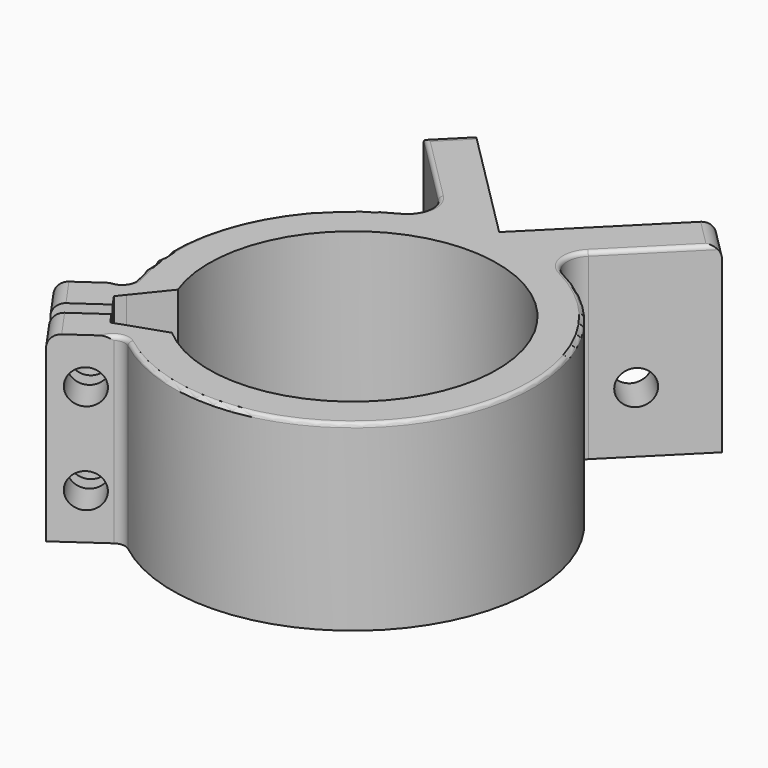
from build123d import *

# Parameters (mm, degrees)
F1_DEPTH      = 45
F2_R          = 4.25
F3_DEPTH      = 10
F4_R          = 4.25
F5_DEPTH      = 10
F6_R          = 4.25
F7_DEPTH      = 22
F9_DEPTH      = 3
F10_R         = 6
F11_T1_DEPTH  = 45
F11_T6_DEPTH  = 45
F11_T11_DEPTH = 50.6773888561
F11_T16_DEPTH = 56.3547777122
F11_T22_DEPTH = 50.6773888561
F11_T24_DEPTH = 24
F11_T26_DEPTH = 24
F11_T28_DEPTH = 25
F11_T30_DEPTH = 25
F12_T3_ANGLE  = 191.1142548037
F12_T6_ANGLE  = 120.6172934525
F12_T9_ANGLE  = 108.2560127517
F12_T12_DEPTH = 25.3616591831
F12_T15_DEPTH = 25.3616591831
F12_T18_ANGLE = 108.2560127517
F12_T21_ANGLE = 120.6172934336
F12_T24_ANGLE = 81.1142548036


# Not quite as in the source:
# - a fillet or chamfer that OpenCascade refuses, or shapes differently, is made with other operations: its cross-section is extruded or revolved along the edge and cut away or added


with BuildPart() as f1:
    # F0 (on Top) → F1 (new body)
    with BuildSketch(Plane.XY):
        with BuildLine():
            Line((29.6984848098, 29.6984848098), (0, 0))
            Line((0, 0), (-29.6984848098, 29.6984848098))
            Line((-29.6984848098, 29.6984848098), (-36.7695526217, 22.627416998))
            Line((-36.7695526217, 22.627416998), (-11.9950181388, -2.1471174849))
            ThreePointArc((-11.9950181388, -2.1471174849), (-39.7071381913, -24.9103714156), (-41.6303752657, -60.7213821032))
            ThreePointArc((-41.6303752657, -60.7213821032), (-40.7005404194, -62.9921096474), (-39.6469587391, -65.2081335788))
            Line((-39.6469587391, -65.2081335788), (-33.2920408775, -57.324366686))
            ThreePointArc((-33.2920408775, -57.324366686), (29.0798975723, -24.6380365095), (-22.9676650232, -72.0691034832))
            Line((-22.9676650232, -72.0691034832), (-32.5494925143, -75.3443658208))
            ThreePointArc((-32.5494925143, -75.3443658208), (-30.8274573358, -77.0923335738), (-29.011693666, -78.7427270775))
            ThreePointArc((-29.011693666, -78.7427270775), (39.2315391454, -66.0032458512), (11.9950181388, -2.1471174849))
            Line((11.9950181388, -2.1471174849), (36.7695526217, 22.627416998))
            Line((36.7695526217, 22.627416998), (29.6984848098, 29.6984848098))
        make_face()
        with BuildLine():
            ThreePointArc((-39.6469587391, -65.2081335788), (-40.7005404194, -62.9921096474), (-41.6303752657, -60.7213821032))
            Line((-41.6303752657, -60.7213821032), (-54.1929009582, -69.517757292))
            Line((-54.1929009582, -69.517757292), (-49.0307130311, -76.8901256906))
            Line((-49.0307130311, -76.8901256906), (-39.1915368437, -70.0006603545))
            Line((-39.1915368437, -70.0006603545), (-41.1990543709, -67.1336281995))
            Line((-41.1990543709, -67.1336281995), (-39.6469587391, -65.2081335788))
        make_face()
        with BuildLine():
            Line((-41.5742193585, -87.5391022664), (-29.011693666, -78.7427270775))
            ThreePointArc((-29.011693666, -78.7427270775), (-30.8274573358, -77.0923335738), (-32.5494925143, -75.3443658208))
            Line((-32.5494925143, -75.3443658208), (-34.8897135711, -76.1443006866))
            Line((-34.8897135711, -76.1443006866), (-36.8972310983, -73.2772685316))
            Line((-36.8972310983, -73.2772685316), (-46.7364072857, -80.1667338678))
            Line((-46.7364072857, -80.1667338678), (-41.5742193585, -87.5391022664))
        make_face()
    extrude(amount=F1_DEPTH)

    # F2 (on face) → F3 (cut, through all)
    with BuildSketch(Plane(origin=(0, 0, 0), x_dir=(-0.7071067812, -0.7071067812, 0), z_dir=(-0.7071067812, 0.7071067812, 0))):
        with Locations((-25.4, 15)):
            Circle(F2_R)
    extrude(amount=-F3_DEPTH, mode=Mode.SUBTRACT)

    # F4 (on face) → F5 (cut, through all)
    with BuildSketch(Plane(origin=(0, 0, 0), x_dir=(-0.7071067812, 0.7071067812, 0), z_dir=(0.7071067812, 0.7071067812, 0))):
        with Locations((25.4, 15)):
            Circle(F4_R)
    extrude(amount=-F5_DEPTH, mode=Mode.SUBTRACT)

    # F6 (on face) → F7 (cut, through all)
    with BuildSketch(Plane(origin=(27.4524247675, -39.206125712, 0), x_dir=(0.8191520443, 0.5735764364, 0), z_dir=(0.5735764364, -0.8191520443, 0))):
        with Locations((-76.5979670285, 33.75)):
            Circle(F6_R)
        with Locations((-76.5979670285, 11.25)):
            Circle(F6_R)
    extrude(amount=-F7_DEPTH, mode=Mode.SUBTRACT)

    # F8 (on face) → F9 (cut)
    with BuildSketch(Plane(origin=(14.8337431678, -21.1847807376, 0), x_dir=(-0.8191520443, -0.5735764364, 0), z_dir=(-0.5735764364, 0.8191520443, 0))):
        Polygon((83.5229670285, 37.7481506141), (76.5979670285, 41.7463012283), (69.6729670285, 37.7481506141), (69.6729670285, 29.7518493859), (76.5979670285, 25.7536987717), (83.5229670285, 29.7518493859), align=None)
        Polygon((76.5979670285, 19.2463012283), (69.6729670285, 15.2481506141), (69.6729670285, 7.2518493859), (76.5979670285, 3.2536987717), (83.5229670285, 7.2518493859), (83.5229670285, 15.2481506141), align=None)
    extrude(amount=-F9_DEPTH, mode=Mode.SUBTRACT)

    # F10
    f10_edges = [f1.edges().sort_by_distance(p)[0] for p in [
        (-11.995018, -2.147117, 22.5),
        (11.995018, -2.147117, 22.5),
    ]]
    fillet(f10_edges, radius=F10_R)

    # F11: fillet of radius 3 on 6 edges, made by hand

    # F11_s2 → F11_t1 (join)
    with BuildSketch(Plane.XY):
        with BuildLine():
            ThreePointArc((-27.3100924069, -80.1341550735), (-29.0764013889, -79.5036829691), (-30.8719515411, -80.0452936647))
            Line((-30.8719515411, -80.0452936647), (-29.011693666, -78.7427270775))
            ThreePointArc((-29.011693666, -78.7427270775), (-28.169485522, -79.4489489742), (-27.3100924069, -80.1341550735))
        make_face()
    extrude(amount=F11_T1_DEPTH)


with BuildPart() as f11_tool4:
    # F11_s5 → F11_t6 (new body)
    with BuildSketch(Plane.XY):
        with BuildLine():
            ThreePointArc((-42.3559079793, -58.6465035538), (-42.3675712465, -60.5219252298), (-43.4906331408, -62.0239486903))
            Line((-43.4906331408, -62.0239486903), (-41.6303752657, -60.7213821032))
            ThreePointArc((-41.6303752657, -60.7213821032), (-42.0059546205, -59.6884232108), (-42.3559079793, -58.6465035538))
        make_face()
    extrude(amount=F11_T6_DEPTH)

    split(bisect_by=Plane(origin=(-57.0727533731, -39.9627721382, 0), x_dir=(0, 0, 1), z_dir=(0.8191520443, 0.5735764364, 0)), keep=Keep.TOP)


with BuildPart() as f1_1:
    add(f1.part)

    # F11_t3: union F11_tool4
    add(f11_tool4.part)


with BuildPart() as f11_tool9:
    # F11_s10 → F11_t11 (new body)
    with BuildSketch(Plane.XY):
        with BuildLine():
            ThreePointArc((-42.3559079793, -58.6465035538), (-42.3675712465, -60.5219252298), (-43.4906331408, -62.0239486903))
            Line((-43.4906331408, -62.0239486903), (-41.6303752657, -60.7213821032))
            ThreePointArc((-41.6303752657, -60.7213821032), (-42.0059546205, -59.6884232108), (-42.3559079793, -58.6465035538))
        make_face()
    extrude(amount=F11_T11_DEPTH)

    split(bisect_by=Plane(origin=(-16.8404428161, -11.7918050066, 35.6081667412), x_dir=(-0.5735764364, 0.8191520443, 0), z_dir=(0.4095760221, 0.2867882182, -0.8660254038)), keep=Keep.TOP)


with BuildPart() as f1_2:
    add(f1_1.part)

    # F11_t8: union F11_tool9
    add(f11_tool9.part)


with BuildPart() as f11_tool14:
    # F11_s15 → F11_t16 (new body)
    with BuildSketch(Plane.XY.offset(-5.6773888561)):
        with BuildLine():
            ThreePointArc((-42.3559079793, -58.6465035538), (-42.3675712465, -60.5219252298), (-43.4906331408, -62.0239486903))
            Line((-43.4906331408, -62.0239486903), (-41.6303752657, -60.7213821032))
            ThreePointArc((-41.6303752657, -60.7213821032), (-42.0059546205, -59.6884232108), (-42.3559079793, -58.6465035538))
        make_face()
    extrude(amount=F11_T16_DEPTH)

    split(bisect_by=Plane(origin=(-24.8212657152, -17.3800373617, 52.4831667412), x_dir=(-0.5735764364, 0.8191520443, 0), z_dir=(0.4095760221, 0.2867882182, -0.8660254038)), keep=Keep.TOP)

    split(bisect_by=Plane(origin=(-8.8596199171, -6.2035726516, -18.7331667412), x_dir=(-0.5735764364, 0.8191520443, 0), z_dir=(0.4095760221, 0.2867882182, 0.8660254038)), keep=Keep.TOP)


with BuildPart() as f1_3:
    add(f1_2.part)

    # F11_t13: union F11_tool14
    add(f11_tool14.part)


with BuildPart() as f11_tool20:
    # F11_s21 → F11_t22 (new body)
    with BuildSketch(Plane.XY.offset(-5.6773888561)):
        with BuildLine():
            ThreePointArc((-42.3559079793, -58.6465035538), (-42.3675712465, -60.5219252298), (-43.4906331408, -62.0239486903))
            Line((-43.4906331408, -62.0239486903), (-41.6303752657, -60.7213821032))
            ThreePointArc((-41.6303752657, -60.7213821032), (-42.0059546205, -59.6884232108), (-42.3559079793, -58.6465035538))
        make_face()
    extrude(amount=F11_T22_DEPTH)

    split(bisect_by=Plane(origin=(-0.878797018, -0.6153402966, -1.8581667412), x_dir=(-0.5735764364, 0.8191520443, 0), z_dir=(0.4095760221, 0.2867882182, 0.8660254038)), keep=Keep.TOP)


with BuildPart() as f1_4:
    add(f1_3.part)

    # F11_t19: union F11_tool20
    add(f11_tool20.part)

    # F11_s25 → F11_t24 (cut)
    with BuildSketch(Plane(origin=(10.5319198952, -15.0411404055, 0), x_dir=(0, 0, 1), z_dir=(0.5735764364, -0.8191520443, 0))):
        with BuildLine():
            ThreePointArc((42, 84.2659730966), (44.1213203436, 83.3872934401), (45, 81.2659730966))
            Line((45, 81.2659730966), (45, 84.2659730966))
            Line((45, 84.2659730966), (42, 84.2659730966))
        make_face()
    extrude(amount=F11_T24_DEPTH, mode=Mode.SUBTRACT)

    # F11_s27 → F11_t26 (cut)
    with BuildSketch(Plane(origin=(17.9884135678, -25.6901169812, 0), x_dir=(0, 0, 1), z_dir=(0.5735764364, -0.8191520443, 0))):
        with BuildLine():
            ThreePointArc((42, 84.2659730966), (44.1213203436, 83.3872934401), (45, 81.2659730966))
            Line((45, 81.2659730966), (45, 84.2659730966))
            Line((45, 84.2659730966), (42, 84.2659730966))
        make_face()
    extrude(amount=F11_T26_DEPTH, mode=Mode.SUBTRACT)

    # F11_s29 → F11_t28 (cut)
    with BuildSketch(Plane(origin=(5.3033008589, 5.3033008589, 0), x_dir=(0, 0, 1), z_dir=(-0.7071067812, -0.7071067812, 0))):
        with BuildLine():
            ThreePointArc((42, 42), (44.1213203436, 41.1213203436), (45, 39))
            Line((45, 39), (45, 42))
            Line((45, 42), (42, 42))
        make_face()
    extrude(amount=F11_T28_DEPTH, mode=Mode.SUBTRACT)

    # F11_s31 → F11_t30 (cut)
    with BuildSketch(Plane(origin=(12.3743686708, -12.3743686708, 0), x_dir=(0, 0, 1), z_dir=(-0.7071067812, 0.7071067812, 0))):
        with BuildLine():
            ThreePointArc((42, 42), (44.1213203436, 41.1213203436), (45, 39))
            Line((45, 39), (45, 42))
            Line((45, 42), (42, 42))
        make_face()
    extrude(amount=F11_T30_DEPTH, mode=Mode.SUBTRACT)

    # F12: fillet of radius 1 on 8 edges, made by hand


with BuildPart() as f12_tool1:
    # F12_s2 → F12_t3 (revolve)
    with BuildSketch(Plane(origin=(21.8044519511, -16.9487951659, 0), x_dir=(0, 0, 1), z_dir=(-0.7895315747, 0.6137099417, 0))):
        with BuildLine():
            ThreePointArc((44, -80.0289208608), (44.7071067812, -79.736027642), (45, -79.0289208608))
            Line((45, -79.0289208608), (45, -80.0289208608))
            Line((45, -80.0289208608), (44, -80.0289208608))
        make_face()
    revolve(axis=Axis((0, -45, 45), (0, 0, 1)), revolution_arc=F12_T3_ANGLE)


with BuildPart() as f12_tool4:
    # F12_s5 → F12_t6 (revolve)
    with BuildSketch(Plane(origin=(21.8044519524, -16.9487951679, 0), x_dir=(0, 0, 1), z_dir=(0.7895315747, -0.6137099417, 0))):
        with BuildLine():
            ThreePointArc((45, 79.0289208601), (44.7071067812, 79.7360276413), (44, 80.0289208601))
            Line((44, 80.0289208601), (45, 80.0289208601))
            Line((45, 80.0289208601), (45, 79.0289208601))
        make_face()
    revolve(axis=Axis((-29.1512222321, -82.5027497974, 45), (0, 0, 1)), revolution_arc=F12_T6_ANGLE)


with BuildPart() as f12_tool7:
    # F12_s8 → F12_t9 (revolve)
    with BuildSketch(Plane(origin=(-11.4115302287, 11.4115302287, 0), x_dir=(0, 0, 1), z_dir=(-0.7071067812, 0.7071067812, 0))):
        with BuildLine():
            ThreePointArc((45, -9), (44.7071067812, -9.7071067812), (44, -10))
            Line((44, -10), (45, -10))
            Line((45, -10), (45, -9))
        make_face()
    revolve(axis=Axis((-22.7252387277, 0.0978217297, 45), (0, 0, -1)), revolution_arc=F12_T9_ANGLE)


with BuildPart() as f12_tool10:
    # F12_s11 → F12_t12 (new body)
    with BuildSketch(Plane(origin=(-29.3449314192, 29.3449314192, 0), x_dir=(0, 0, 1), z_dir=(0.7071067812, -0.7071067812, 0))):
        with BuildLine():
            ThreePointArc((45, 9), (44.7071067812, 9.7071067812), (44, 10))
            Line((44, 10), (45, 10))
            Line((45, 10), (45, 9))
        make_face()
    extrude(amount=F12_T12_DEPTH)


with BuildPart() as f12_tool13:
    # F12_s14 → F12_t15 (new body)
    with BuildSketch(Plane(origin=(11.4115302287, 11.4115302287, 0), x_dir=(0, 0, 1), z_dir=(0.7071067812, 0.7071067812, 0))):
        with BuildLine():
            ThreePointArc((45, 9), (44.7071067812, 9.7071067812), (44, 10))
            Line((44, 10), (45, 10))
            Line((45, 10), (45, 9))
        make_face()
    extrude(amount=F12_T15_DEPTH)


with BuildPart() as f12_tool16:
    # F12_s17 → F12_t18 (revolve)
    with BuildSketch(Plane(origin=(18.0839699719, -9.1126914559, 0), x_dir=(0, 0, 1), z_dir=(0.8930261729, -0.4500047273, 0))):
        with BuildLine():
            ThreePointArc((44, -4.313822221), (44.7071067812, -4.0209290022), (45, -3.313822221))
            Line((45, -3.313822221), (45, -4.313822221))
            Line((45, -4.313822221), (44, -4.313822221))
        make_face()
    revolve(axis=Axis((22.7252387277, 0.0978217298, 45), (0, 0, -1)), revolution_arc=F12_T18_ANGLE)


with BuildPart() as f12_tool19:
    # F12_s20 → F12_t21 (revolve)
    with BuildSketch(Plane(origin=(13.1349335644, -40.7681011714, 0), x_dir=(0, 0, 1), z_dir=(-0.3066630011, 0.9518181569, 0))):
        with BuildLine():
            ThreePointArc((45, -57.299835051), (44.7071067812, -58.0069418322), (44, -58.299835051))
            Line((44, -58.299835051), (45, -58.299835051))
            Line((45, -58.299835051), (45, -57.299835051))
        make_face()
    revolve(axis=Axis((-45.2113624502, -59.5664925573, 45), (0, 0, -1)), revolution_arc=F12_T21_ANGLE)


with BuildPart() as f12_tool22:
    # F12_s23 → F12_t24 (revolve)
    with BuildSketch(Plane(origin=(-18.0839699719, -9.1126914559, 0), x_dir=(0, 0, 1), z_dir=(0.8930261729, 0.4500047273, 0))):
        with BuildLine():
            ThreePointArc((45, -3.313822221), (44.7071067812, -4.0209290022), (44, -4.313822221))
            Line((44, -4.313822221), (45, -4.313822221))
            Line((45, -4.313822221), (45, -3.313822221))
        make_face()
    revolve(axis=Axis((0, -45, 45), (0, 0, 1)), revolution_arc=F12_T24_ANGLE)


with BuildPart() as f1_5:
    add(f1_4.part)

    # F12_t25: cut F12_tool1, F12_tool4, F12_tool7, F12_tool10, F12_tool13, F12_tool16, F12_tool19, F12_tool22
    add([f12_tool1.part, f12_tool4.part, f12_tool7.part, f12_tool10.part, f12_tool13.part, f12_tool16.part, f12_tool19.part, f12_tool22.part], mode=Mode.SUBTRACT)


solid = f1_5.part
